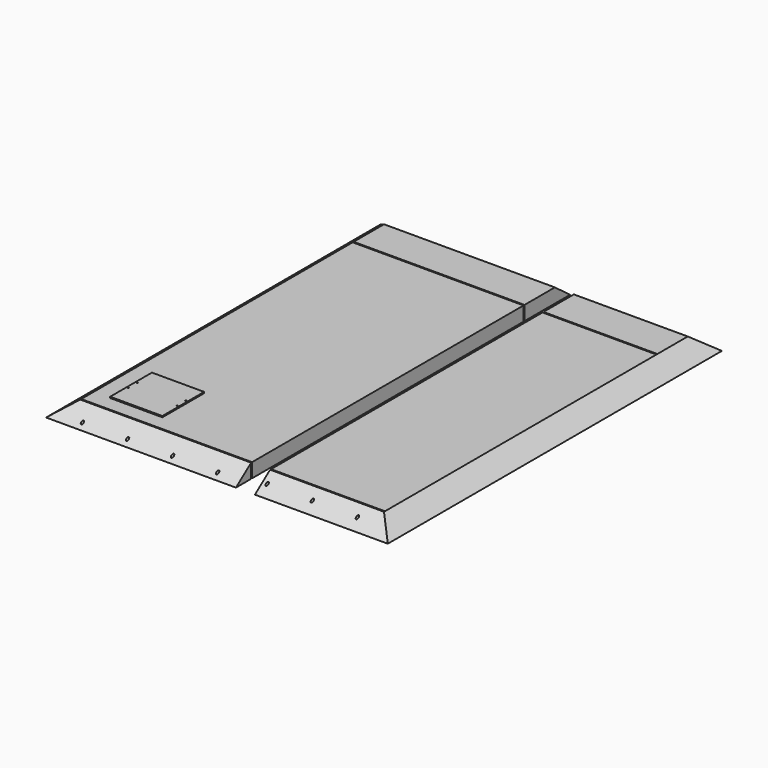
from build123d import *

# Parameters (mm, degrees)
F0_W           = 457.2
F0_H           = 1117.6
F1_DEPTH       = 38.1
F2_SIZE        = 38.09999
F3_W           = 50.8
F3_H           = 50.8
F4_DEPTH       = 406.4
F4_DEPTH_BACK  = 406.4
F5_W           = 203.2
F5_H           = 152.4
F6_DEPTH       = 25.4
F8_DEPTH       = 38.1
F0_W_2         = 304.8
F10_DEPTH      = 1117.6
F11_DEPTH      = 1117.6
F13_DEPTH      = 1117.6
F14_W          = 127
F14_H          = 127
F15_DEPTH      = 19.05
F16_R          = 6.35
F17_DEPTH      = 25.4
F18_R          = 3.175
F19_DEPTH      = 101.601
F20_W          = 139.7
F20_H          = 139.7
F20_W_2        = 127
F20_H_2        = 127
F21_DEPTH      = 3.175
F22_R          = 1.651
F23_DEPTH      = 3.175
F25_SIZE2      = 50.79999
F25_SIZE       = 38.09999
F25_2_SIZE2    = 50.79999
F25_2_SIZE     = 38.09999
F25_3_SIZE2    = 50.79999
F25_3_SIZE     = 38.09999
F25_4_SIZE2    = 50.79999
F25_4_SIZE     = 38.09999
F26_W          = 457.2
F26_H          = 3.175
F27_DEPTH      = 38.101
F28_DEPTH      = 38.101
F29_W          = 304.8
F29_H          = 3.175
F30_DEPTH      = 25.4
F31_R          = 3.175
F32_DEPTH      = 558.801
F32_DEPTH_BACK = 558.801
F33_R          = 3.175
F34_DEPTH      = 558.801
F34_DEPTH_BACK = 558.801


# Not quite as in the source:
# - a fillet or chamfer is up to 0.001 mm smaller than in the source, because OpenCascade refuses the exact size
# - ends of sketch curves that miss each other by under 0.0002 mm in the source are joined


with BuildPart() as f1:
    # F0 (on Top) → F1 (new body)
    with BuildSketch(Plane.XY):
        with Locations((-177.8, 0)):
            Rectangle(F0_W, F0_H)
    extrude(amount=F1_DEPTH)

    # F2 (size 38.1 in the source; OpenCascade refuses exactly that, so slightly less here)
    f2_edges = [f1.edges().sort_by_distance(p)[0] for p in [
        (-177.8, -558.8, 38.1),
        (-177.8, 558.8, 38.1),
    ]]
    chamfer(f2_edges, length=F2_SIZE)

    # F3 (on Front) → F4 (cut, two sides)
    with BuildSketch(Plane.XZ) as f4_sk:
        with Locations((114.3, 25.4)):
            Rectangle(F3_W, F3_H)
    extrude(amount=-F4_DEPTH, mode=Mode.SUBTRACT)
    extrude(f4_sk.sketch, amount=F4_DEPTH_BACK, mode=Mode.SUBTRACT)

    # F5 (on face) → F6 (cut)
    with BuildSketch(Plane.XY.offset(38.1)):
        with Locations((-266.7, -444.5)):
            Rectangle(F5_W, F5_H)
    extrude(amount=-F6_DEPTH, mode=Mode.SUBTRACT)


with BuildPart() as f8:
    # F0 (on Top) → F8 (new body)
    with BuildSketch(Plane.XY):
        with Locations((-177.8, 0)):
            Rectangle(F0_W, F0_H)
    extrude(amount=F8_DEPTH)

    # F12 (on face) → F13 (join, through all)
    with BuildSketch(Plane.XZ.offset(558.8)):
        Polygon((50.8, 38.1), (-406.4, 38.1), (-457.2, 0), (-406.4, 0), (50.8, 0), align=None)
    extrude(amount=-F13_DEPTH)

    # F14 (on face) → F15 (cut)
    with BuildSketch(Plane.XY.offset(38.1)):
        with Locations((-292.1, -393.7)):
            Rectangle(F14_W, F14_H)
    extrude(amount=-F15_DEPTH, mode=Mode.SUBTRACT)

    # F16 (on face) → F17 (cut)
    with BuildSketch(Plane.XY.offset(19.05)):
        with Locations((-260.35, -431.8)):
            Circle(F16_R)
    extrude(amount=-F17_DEPTH, mode=Mode.SUBTRACT)

    # F18 (on face) → F19 (cut, through all)
    with BuildSketch(Plane.YZ.offset(-355.6)):
        with Locations((-431.8, 25.4)):
            Circle(F18_R)
    extrude(amount=-F19_DEPTH, mode=Mode.SUBTRACT)

    # F25 (size 38.1 and 50.8 in the source; OpenCascade refuses exactly that, so slightly less here)
    f25_edges = [f8.edges().sort_by_distance(p)[0] for p in [
        (-177.8, 558.8, 38.1),
    ]]
    f25_side = f8.faces().sort_by_distance((-190.722807, 558.8, 18.715789))[0]
    chamfer(f25_edges, length=F25_SIZE, length2=F25_SIZE2, reference=f25_side)

    # F25#2 (size 38.1 and 50.8 in the source; OpenCascade refuses exactly that, so slightly less here)
    f25_2_edges = [f8.edges().sort_by_distance(p)[0] for p in [
        (-177.8, -558.8, 38.1),
    ]]
    f25_2_side = f8.faces().sort_by_distance((-190.722807, -558.8, 18.715789))[0]
    chamfer(f25_2_edges, length=F25_2_SIZE, length2=F25_2_SIZE2, reference=f25_2_side)

    # F26 (on face) → F27 (cut, through all)
    with BuildSketch(Plane.XY.offset(38.1)):
        with Locations((-177.8, -506.4125)):
            Rectangle(F26_W, F26_H)
        with Locations((-177.8, 404.8125)):
            Rectangle(F26_W, F26_H)
    extrude(amount=-F27_DEPTH, mode=Mode.SUBTRACT)

    # F26 (on face) → F28 (cut, through all)
    with BuildSketch(Plane.XY.offset(38.1)):
        with Locations((-177.8, -506.4125)):
            Rectangle(F26_W, F26_H)
        with Locations((-177.8, 404.8125)):
            Rectangle(F26_W, F26_H)
    extrude(amount=-F28_DEPTH, mode=Mode.SUBTRACT)

    # F33 (on Front) → F34 (cut, two sides)
    with BuildSketch(Plane.XZ) as f34_sk:
        with Locations((-9.2376703805, 10.6194233916)):
            Circle(F33_R)
        with Locations((-129.8876703805, 10.6194233916)):
            Circle(F33_R)
        with Locations((-250.5376703805, 10.6194233916)):
            Circle(F33_R)
        with Locations((-371.1876703805, 10.6194233916)):
            Circle(F33_R)
    extrude(amount=F34_DEPTH, mode=Mode.SUBTRACT)
    extrude(f34_sk.sketch, amount=-F34_DEPTH_BACK, mode=Mode.SUBTRACT)


with BuildPart() as f8b:
    # F0 (on Top) → F8, piece 2 (new body)
    with BuildSketch(Plane.XY):
        with Locations((254, 0)):
            Rectangle(F0_W_2, F0_H)
    extrude(amount=F8_DEPTH)

    # F9 (on face) → F10 (join, through all)
    with BuildSketch(Plane.XZ.offset(558.8)):
        Polygon((457.2, 0), (406.4, 38.1), (406.4, 0), align=None)
    extrude(amount=-F10_DEPTH)

    # F9 (on face) → F11 (join, through all)
    with BuildSketch(Plane.XZ.offset(558.8)):
        Polygon((457.2, 0), (406.4, 38.1), (101.6, 38.1), (101.6, 0), (406.4, 0), align=None)
    extrude(amount=-F11_DEPTH)

    # F25#3 (size 38.1 and 50.8 in the source; OpenCascade refuses exactly that, so slightly less here)
    f25_3_edges = [f8b.edges().sort_by_distance(p)[0] for p in [
        (254, 558.8, 38.1),
    ]]
    f25_3_side = f8b.faces().sort_by_distance((267.025641, 558.8, 18.561538))[0]
    chamfer(f25_3_edges, length=F25_3_SIZE, length2=F25_3_SIZE2, reference=f25_3_side)

    # F25#4 (size 38.1 and 50.8 in the source; OpenCascade refuses exactly that, so slightly less here)
    f25_4_edges = [f8b.edges().sort_by_distance(p)[0] for p in [
        (254, -558.8, 38.1),
    ]]
    f25_4_side = f8b.faces().sort_by_distance((267.025641, -558.8, 18.561538))[0]
    chamfer(f25_4_edges, length=F25_4_SIZE, length2=F25_4_SIZE2, reference=f25_4_side)

    # F29 (on face) → F30 (cut)
    with BuildSketch(Plane.XY.offset(38.1)):
        with Locations((254, -506.4125)):
            Rectangle(F29_W, F29_H)
        with Locations((254, 404.8125)):
            Rectangle(F29_W, F29_H)
    extrude(amount=-F30_DEPTH, mode=Mode.SUBTRACT)

    # F31 (on Front) → F32 (cut, two sides)
    with BuildSketch(Plane.XZ) as f32_sk:
        with Locations((355.6, 19.05)):
            Circle(F31_R)
        with Locations((234.95, 19.05)):
            Circle(F31_R)
        with Locations((114.3, 19.05)):
            Circle(F31_R)
    extrude(amount=-F32_DEPTH, mode=Mode.SUBTRACT)
    extrude(f32_sk.sketch, amount=F32_DEPTH_BACK, mode=Mode.SUBTRACT)


with BuildPart() as f21:
    # F20 (on face) → F21 (new body)
    with BuildSketch(Plane.XY.offset(38.1)):
        with Locations((-292.1, -393.7)):
            Rectangle(F20_W, F20_H)
        with Locations((-292.1, -393.7)):
            Rectangle(F20_W_2, F20_H_2, mode=Mode.SUBTRACT)
        with Locations((-292.1, -393.7)):
            Rectangle(F20_W_2, F20_H_2)
    extrude(amount=F21_DEPTH)

    # F22 (on face) → F23 (cut, through all)
    with BuildSketch(Plane.XY.offset(41.275)):
        with Locations((-357.5131893158, -408.5888405323)):
            Circle(F22_R)
        with Locations((-226.6868106842, -408.5888405323)):
            Circle(F22_R)
        with Locations((-226.6868106842, -378.8111594677)):
            Circle(F22_R)
        with Locations((-357.5131893158, -378.8111594677)):
            Circle(F22_R)
    extrude(amount=-F23_DEPTH, mode=Mode.SUBTRACT)


solid = Compound([f8.part, f8b.part, f21.part])
